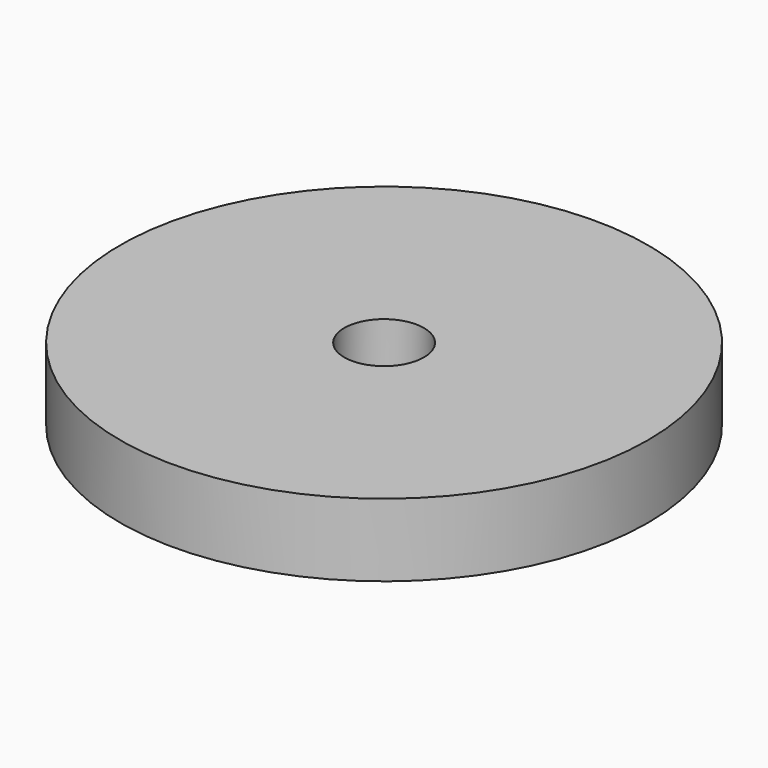
from build123d import *

# Parameters (mm, degrees)
F0_R     = 23.1307530626
F0_R_2   = 3.4880603878
F1_DEPTH = 6.3754
F0_R_3   = 3.1113947691
F2_DEPTH = 2.9718


with BuildPart() as f1:
    # F0 (on Top) → F1 (new body)
    with BuildSketch(Plane.XY):
        Circle(F0_R)
        Circle(F0_R_2, mode=Mode.SUBTRACT)
    extrude(amount=F1_DEPTH)


with BuildPart() as f2:
    # F0 (on Top) → F2 (new body)
    with BuildSketch(Plane.XY):
        Circle(F0_R_3)
    extrude(amount=-F2_DEPTH)


solid = Compound([f1.part, f2.part])
